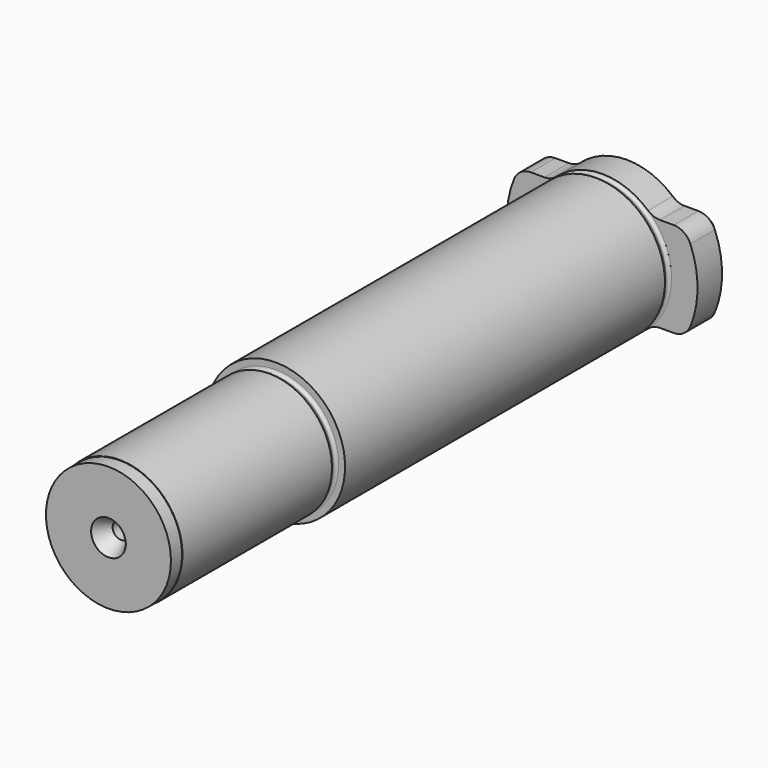
from build123d import *

# Parameters (mm, degrees)
F0_R            = 11.4427
F1_DEPTH        = 2.54
F2_R            = 11.52271
F3_DEPTH        = 35.7378
F4_R            = 12.7
F4_R_2          = 11.52271
F5_DEPTH        = 74.7268
F7_DEPTH        = 7.1374
F8_T1_DEPTH     = 7.1374
F8_T3_DEPTH     = 18.5145836873
F9_SIZE         = 1.524
F13_D           = 3.048
F13_DEPTH       = 12.7
F13_CSINK_D     = 6.35
F13_CSINK_ANGLE = 60
F13_TIP         = 0.9157115834
F15_D           = 3.048
F15_DEPTH       = 12.7
F15_CSINK_D     = 6.35
F15_CSINK_ANGLE = 60
F15_TIP         = 0.9157115834


# Not quite as in the source:
# - a fillet or chamfer that OpenCascade refuses, or shapes differently, is made with other operations: its cross-section is extruded or revolved along the edge and cut away or added


with BuildPart() as f1:
    # F0 (on Front) → F1 (new body)
    with BuildSketch(Plane.XZ):
        Circle(F0_R)
    extrude(amount=-F1_DEPTH)

    # F2 (on face) → F3 (join)
    with BuildSketch(Plane(origin=(0, 2.54, 0), x_dir=(-1, 0, 0), z_dir=(0, 1, 0))):
        Circle(F2_R)
    extrude(amount=F3_DEPTH)

    # F4 (on face) → F5 (join)
    with BuildSketch(Plane(origin=(0, 38.2778, 0), x_dir=(-1, 0, 0), z_dir=(0, 1, 0))):
        Circle(F4_R)
        Circle(F4_R_2, mode=Mode.SUBTRACT)
        Circle(F4_R_2)
    extrude(amount=F5_DEPTH)

    # F6 (on face) → F7 (join)
    with BuildSketch(Plane(origin=(0, 113.0046, 0), x_dir=(-1, 0, 0), z_dir=(0, 1, 0))):
        with BuildLine():
            ThreePointArc((12.7, 0), (11.8067080769, 4.678850755), (9.2524969468, 8.6995))
            ThreePointArc((9.2524969468, 8.6995), (0, 12.7), (-9.2524969468, 8.6995))
            ThreePointArc((-9.2524969468, 8.6995), (-12.7, 0), (-9.2524969468, -8.6995))
            ThreePointArc((-9.2524969468, -8.6995), (0, -12.7), (9.2524969468, -8.6995))
            ThreePointArc((9.2524969468, -8.6995), (11.8067080769, -4.678850755), (12.7, 0))
        make_face()
        with BuildLine():
            ThreePointArc((15.126606354, -8.6995), (17.4498, 0), (15.126606354, 8.6995))
            Line((15.126606354, 8.6995), (9.2524969468, 8.6995))
            ThreePointArc((9.2524969468, 8.6995), (11.8067080769, 4.678850755), (12.7, 0))
            ThreePointArc((12.7, 0), (11.8067080769, -4.678850755), (9.2524969468, -8.6995))
            Line((9.2524969468, -8.6995), (15.126606354, -8.6995))
        make_face()
        with BuildLine():
            ThreePointArc((-9.2524969468, -8.6995), (-12.7, 0), (-9.2524969468, 8.6995))
            Line((-9.2524969468, 8.6995), (-15.126606354, 8.6995))
            ThreePointArc((-15.126606354, 8.6995), (-17.4498, 0), (-15.126606354, -8.6995))
            Line((-15.126606354, -8.6995), (-9.2524969468, -8.6995))
        make_face()
    extrude(amount=F7_DEPTH)

    # F8: fillet of radius 3.302 on 8 edges, made by hand

    # F8_s2 → F8_t1 (join)
    with BuildSketch(Plane.XZ.offset(-120.142)):
        with BuildLine():
            ThreePointArc((-8.4002604126, -9.525), (-9.4168948242, -8.9127618272), (-10.5843281199, -8.6995))
            Line((-10.5843281199, -8.6995), (-9.2524969468, -8.6995))
            ThreePointArc((-9.2524969468, -8.6995), (-8.8360241715, -9.1222078928), (-8.4002604126, -9.525))
        make_face()
        with BuildLine():
            ThreePointArc((8.4002604126, -9.525), (9.4168948242, -8.9127618272), (10.5843281199, -8.6995))
            Line((10.5843281199, -8.6995), (9.2524969468, -8.6995))
            ThreePointArc((9.2524969468, -8.6995), (8.8360241715, -9.1222078928), (8.4002604126, -9.525))
        make_face()
        with BuildLine():
            ThreePointArc((-8.4002604126, 9.525), (-9.4168948242, 8.9127618272), (-10.5843281199, 8.6995))
            Line((-10.5843281199, 8.6995), (-9.2524969468, 8.6995))
            ThreePointArc((-9.2524969468, 8.6995), (-8.8360241715, 9.1222078928), (-8.4002604126, 9.525))
        make_face()
        with BuildLine():
            ThreePointArc((8.4002604126, 9.525), (9.4168948242, 8.9127618272), (10.5843281199, 8.6995))
            Line((10.5843281199, 8.6995), (9.2524969468, 8.6995))
            ThreePointArc((9.2524969468, 8.6995), (8.8360241715, 9.1222078928), (8.4002604126, 9.525))
        make_face()
    extrude(amount=F8_T1_DEPTH)

    # F8_s4 → F8_t3 (cut)
    with BuildSketch(Plane.XZ.offset(-125.8305918437)):
        with BuildLine():
            ThreePointArc((-13.0777382827, -8.6995), (-14.913976773, -8.1418454969), (-16.1299931781, -6.6572396768))
            ThreePointArc((-16.1299931781, -6.6572396768), (-15.6616238106, -7.6947423385), (-15.126606354, -8.6995))
            Line((-15.126606354, -8.6995), (-13.0777382827, -8.6995))
        make_face()
        with BuildLine():
            ThreePointArc((13.0777382827, -8.6995), (14.913976773, -8.1418454969), (16.1299931781, -6.6572396768))
            ThreePointArc((16.1299931781, -6.6572396768), (15.6616238106, -7.6947423385), (15.126606354, -8.6995))
            Line((15.126606354, -8.6995), (13.0777382827, -8.6995))
        make_face()
        with BuildLine():
            ThreePointArc((-16.1299931781, 6.6572396768), (-14.913976773, 8.1418454969), (-13.0777382827, 8.6995))
            Line((-13.0777382827, 8.6995), (-15.126606354, 8.6995))
            ThreePointArc((-15.126606354, 8.6995), (-15.6616238106, 7.6947423385), (-16.1299931781, 6.6572396768))
        make_face()
        with BuildLine():
            ThreePointArc((16.1299931781, 6.6572396768), (14.913976773, 8.1418454969), (13.0777382827, 8.6995))
            Line((13.0777382827, 8.6995), (15.126606354, 8.6995))
            ThreePointArc((15.126606354, 8.6995), (15.6616238106, 7.6947423385), (16.1299931781, 6.6572396768))
        make_face()
    extrude(amount=F8_T3_DEPTH, mode=Mode.SUBTRACT)

    # F9
    f9_edges = [f1.edges().sort_by_distance(p)[0] for p in [
        (0, 120.142, 12.7),
        (0, 120.142, -12.7),
        (-9.416895, 120.142, -8.912762),
        (9.416895, 120.142, -8.912762),
        (11.831033, 120.142, -8.6995),
        (14.913977, 120.142, -8.141845),
        (17.4498, 120.142, 0),
        (14.913977, 120.142, 8.141845),
        (11.831033, 120.142, 8.6995),
        (9.416895, 120.142, 8.912762),
        (-9.416895, 120.142, 8.912762),
        (-11.831033, 120.142, 8.6995),
        (-14.913977, 120.142, 8.141845),
        (-17.4498, 120.142, 0),
        (-14.913977, 120.142, -8.141845),
        (-11.831033, 120.142, -8.6995),
    ]]
    chamfer(f9_edges, length=F9_SIZE)

    # F10 (on Top) → F11 (revolve, cut)
    with BuildSketch(Plane.XY):
        with BuildLine():
            Line((-12.7, 113.0046), (-12.7, 111.4806))
            Line((-12.7, 111.4806), (-12.2600590949, 112.2426))
            ThreePointArc((-12.2600590949, 112.2426), (-12.2600590949, 112.7506), (-12.7, 113.0046))
        make_face()
        with BuildLine():
            Line((11.52271, 36.7538), (11.52271, 38.2778))
            ThreePointArc((11.52271, 38.2778), (11.0827690949, 38.0238), (11.0827690949, 37.5158))
            Line((11.0827690949, 37.5158), (11.52271, 36.7538))
        make_face()
    revolve(axis=Axis((0, 32.0415347815, 0), (0, 1, 0)), mode=Mode.SUBTRACT)

    # F13
    with Locations(Plane.XZ):
        with Locations((0, 0)):
            CounterSinkHole(F13_D / 2, F13_CSINK_D / 2, depth=F13_DEPTH, counter_sink_angle=F13_CSINK_ANGLE)
            with Locations((0, 0, -(F13_DEPTH + F13_TIP / 2))):  # 118° drill point
                Cone(0, F13_D / 2, F13_TIP, mode=Mode.SUBTRACT)

    # F15
    with Locations(Plane(origin=(0, 120.142, 0), x_dir=(-1, 0, 0), z_dir=(0, 1, 0))):
        with Locations((0, 0)):
            CounterSinkHole(F15_D / 2, F15_CSINK_D / 2, depth=F15_DEPTH, counter_sink_angle=F15_CSINK_ANGLE)
            with Locations((0, 0, -(F15_DEPTH + F15_TIP / 2))):  # 118° drill point
                Cone(0, F15_D / 2, F15_TIP, mode=Mode.SUBTRACT)


solid = f1.part
